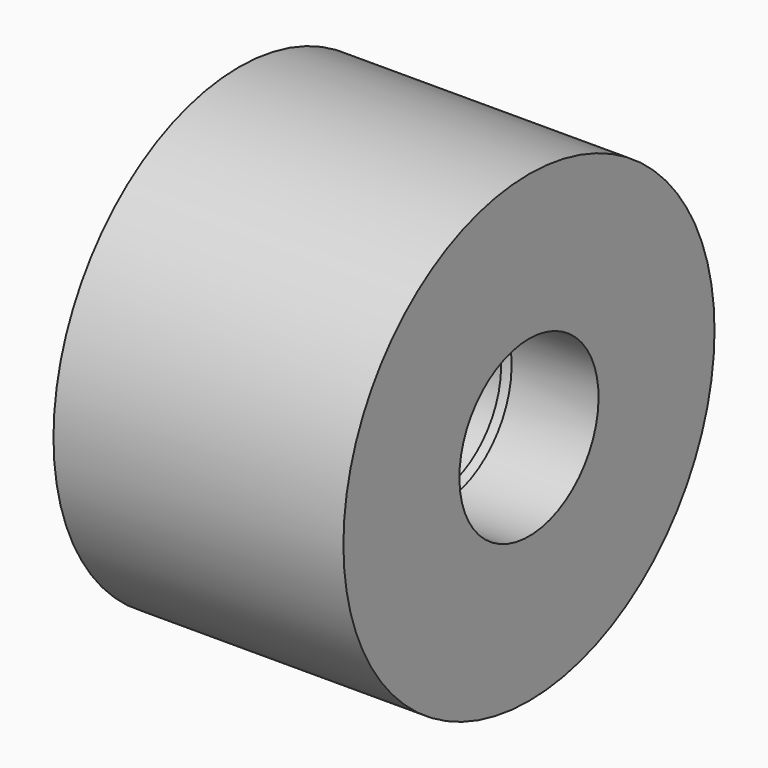
from build123d import *

# Parameters (mm, degrees)
F0_W    = 40
F0_H    = 15
F2_SIZE = 0.99999


# Not quite as in the source:
# - a fillet or chamfer is up to 0.001 mm smaller than in the source, because OpenCascade refuses the exact size


with BuildPart() as f1:
    # F0 (on Front) → F1 (revolve)
    with BuildSketch(Plane.XZ):
        Polygon((-45, 40), (-50, 40), (-50, 14), (-40, 14), (-40, 12.5), (-25, 12.5), (-25, 14), (-15, 14), (-15, 15), (0, 15), (0, 40), (-5, 40), (-5, 25), (-45, 25), align=None)
        with Locations((-25, 32.5)):
            Rectangle(F0_W, F0_H)
    revolve(axis=Axis((-17.5871104002, 0, 0), (1, 0, 0)))

    # F2 (size 1 in the source; OpenCascade refuses exactly that, so slightly less here)
    f2_edges = [f1.edges().sort_by_distance(p)[0] for p in [
        (-15, 0, -14),
        (-50, 0, -14),
    ]]
    chamfer(f2_edges, length=F2_SIZE)


solid = f1.part
